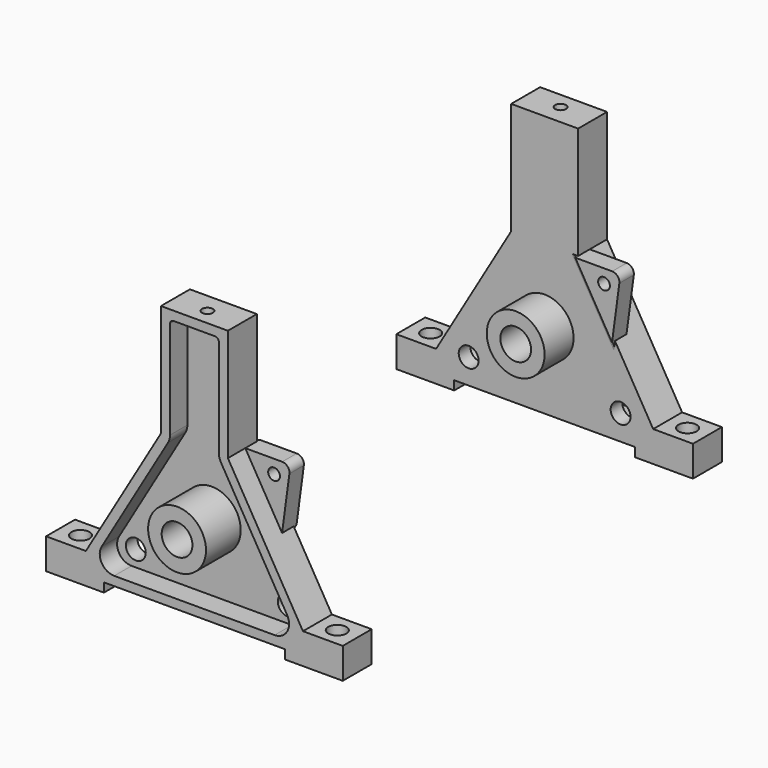
from build123d import *

# Parameters (mm, degrees)
F1_DEPTH       = 20
F4_DEPTH       = 12
F5_R           = 5.5
F6_DEPTH       = 25
F7_R           = 16
F7_R_2         = 8.5
F8_DEPTH       = 24
F9_R           = 16
F9_R_2         = 8.5
F10_DEPTH      = 20
F11_R          = 5
F12_DEPTH      = 25
F13_R          = 3
F14_DEPTH      = 10
F16_R          = 3.25
F17_DEPTH      = 8
F17_DEPTH_BACK = 2
F18_T4_DEPTH   = 54.3641994781


# Not quite as in the source:
# - a fillet or chamfer that OpenCascade refuses, or shapes differently, is made with other operations: its cross-section is extruded or revolved along the edge and cut away or added


with BuildPart() as f1:
    # F0 (on Front) → F1 (new body)
    with BuildSketch(Plane.XZ):
        Polygon((0, 149.7230514048), (-18.5, 149.7230514048), (-18.5, 87.7230514048), (-60, 17), (-82, 17), (-82, 0), (-50, 0), (-50, 5), (0, 5), align=None)
    extrude(amount=F1_DEPTH)

    # F2: F1 across plane


with BuildPart() as f1_1:
    add(f1.part)
    add(f1.part.mirror(Plane.YZ))

    # F3 (on face) → F4 (cut)
    with BuildSketch(Plane.XZ.offset(20)):
        with BuildLine():
            ThreePointArc((44.3403253904, 9.9999997765), (51.2825960529, 14.0244648378), (51.2401352836, 22.0487802643))
            Line((51.2401352836, 22.0487802643), (14.6001903304, 84.489472081))
            ThreePointArc((14.6001903304, 84.489472081), (13.7799458472, 86.4404536205), (13.5000002235, 88.5382525688))
            Line((13.5000002235, 88.5382525688), (13.5000002235, 142.7230516283))
            ThreePointArc((13.5000002235, 142.7230516283), (12.9142137859, 144.1372651906), (11.5000002235, 144.7230516283))
            Line((11.5000002235, 144.7230516283), (-11.5000002235, 144.7230516283))
            ThreePointArc((-11.5000002235, 144.7230516283), (-12.9142137859, 144.1372651906), (-13.5000002235, 142.7230516283))
            Line((-13.5000002235, 142.7230516283), (-13.5000002235, 88.5382525688))
            ThreePointArc((-13.5000002235, 88.5382525688), (-13.7799458472, 86.4404536205), (-14.6001903304, 84.489472081))
            Line((-14.6001903304, 84.489472081), (-51.2401352836, 22.0487802643))
            ThreePointArc((-51.2401352836, 22.0487802643), (-51.2825960529, 14.0244648378), (-44.3403253904, 9.9999997765))
            Line((-44.3403253904, 9.9999997765), (44.3403253904, 9.9999997765))
        make_face()
    extrude(amount=-F4_DEPTH, mode=Mode.SUBTRACT)

    # F5 (on face) → F6 (cut)
    with BuildSketch(Plane.XZ.offset(8)):
        with Locations((-42, 18.8791340478)):
            Circle(F5_R)
        with Locations((42, 18.8791340478)):
            Circle(F5_R)
    extrude(amount=-F6_DEPTH, mode=Mode.SUBTRACT)

    # F7 (on face) → F8 (join)
    with BuildSketch(Plane.XZ.offset(8)):
        with Locations((0, 46.9999997765)):
            Circle(F7_R)
        with Locations((0, 46.9999997765)):
            Circle(F7_R_2, mode=Mode.SUBTRACT)
    extrude(amount=F8_DEPTH)

    # F9 (on face) → F10 (join)
    with BuildSketch(Plane(origin=(0, 0, 0), x_dir=(-1, 0, 0), z_dir=(0, 1, 0))):
        with Locations((0, 46.9999997765)):
            Circle(F9_R)
        with Locations((0, 46.9999997765)):
            Circle(F9_R_2, mode=Mode.SUBTRACT)
    extrude(amount=F10_DEPTH)

    # F11 (on face) → F12 (cut)
    with BuildSketch(Plane.XY.offset(17)):
        with Locations((-71, -10)):
            Circle(F11_R)
        with Locations((71, -10)):
            Circle(F11_R)
    extrude(amount=-F12_DEPTH, mode=Mode.SUBTRACT)

    # F13 (on face) → F14 (cut)
    with BuildSketch(Plane.XY.offset(149.7230514048)):
        with Locations((0, -11)):
            Circle(F13_R)
    extrude(amount=-F14_DEPTH, mode=Mode.SUBTRACT)

    # F16 (on face) → F17 (join, two sides)
    with BuildSketch(Plane(origin=(0, 0, 0), x_dir=(-1, 0, 0), z_dir=(0, 1, 0))) as f17_sk:
        with BuildLine():
            Line((-38.8562884141, 53.0324771416), (-18.5, 87.7230514048))
            Line((-18.5, 87.7230514048), (-38.9288780249, 87.7230514048))
            ThreePointArc((-38.9288780249, 87.7230514048), (-41.9390972513, 86.3571698928), (-42.8935150835, 83.1923415092))
            Line((-42.8935150835, 83.1923415092), (-38.8562884141, 53.0324771416))
        make_face()
        with Locations((-34.4246865011, 80.2230514048)):
            Circle(F16_R, mode=Mode.SUBTRACT)
    extrude(amount=-F17_DEPTH)
    extrude(f17_sk.sketch, amount=F17_DEPTH_BACK)

    # F18: fillet of radius 3 on 1 edges, made by hand


with BuildPart() as f18_tool2:
    # F18_s3 → F18_t4 (new body)
    with BuildSketch(Plane(origin=(-37.1310167355, 0, 63.2775615735), x_dir=(0, 1, 0), z_dir=(0.506097561, 0, -0.8624762366))):
        with BuildLine():
            ThreePointArc((2, 60.3522327352), (0.5505102572, 59.255856418), (0, 57.5238056104))
            Line((0, 57.5238056104), (0, 60.3522327352))
            Line((0, 60.3522327352), (2, 60.3522327352))
        make_face()
    extrude(amount=F18_T4_DEPTH)

    split(bisect_by=Plane(origin=(31.1982792576, 0, -4.176229824), x_dir=(0, 1, 0), z_dir=(-0.9911592647, 0, 0.1326774739)), keep=Keep.TOP)

    split(bisect_by=Plane.XY.offset(87.7230514048), keep=Keep.BOTTOM)


with BuildPart() as f1_2:
    add(f1_1.part)

    # F18_t1: union F18_tool2
    add(f18_tool2.part)


with BuildPart() as f19_1:
    # F19: instance of F1
    add(f1_2.part.mirror(Plane(origin=(0, 111, 55.7488868878), x_dir=(-1, 0, 0), z_dir=(0, 1, 0))))


solid = Compound([f1_2.part, f19_1.part])
